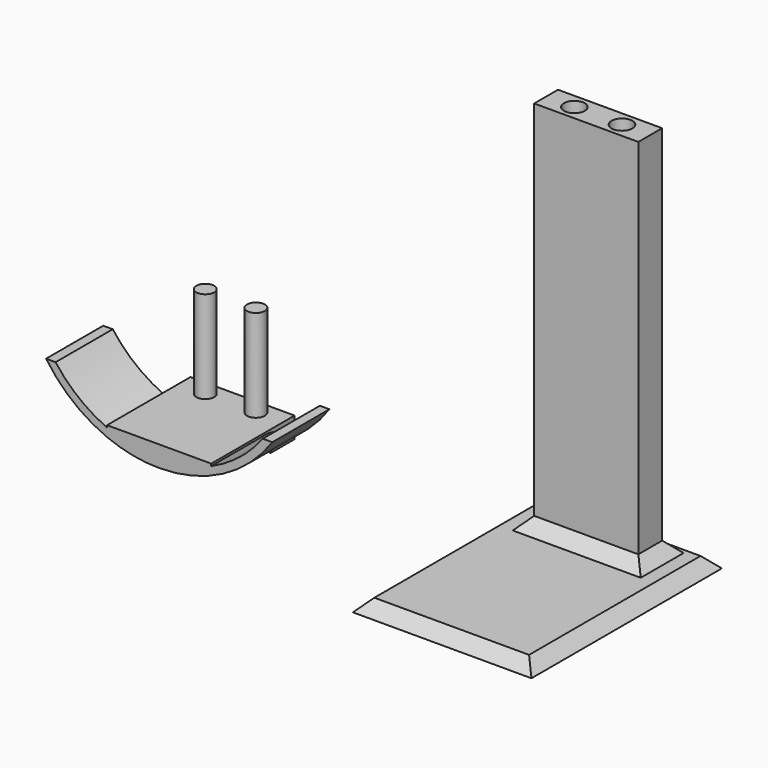
from build123d import *

# Parameters (mm, degrees)
F0_W      = 76.2
F0_H      = 101.6
F0_W_2    = 44.45
F0_H_2    = 12.7
F1_DEPTH  = 5.08
F2_DEPTH  = 165.1
F3_R      = 4.445
F4_DEPTH  = 50.8
F5_W      = 44.45
F5_H      = 12.7
F5_R      = 3.81
F6_DEPTH  = 8.89
F7_DEPTH  = 48.26
F9_DEPTH  = 31.75
F10_DEPTH = 1.27
F11_SIZE  = 5.07999


# Not quite as in the source:
# - a fillet or chamfer is up to 0.001 mm smaller than in the source, because OpenCascade refuses the exact size


with BuildPart() as f1:
    # F0 (on Top) → F1 (new body)
    with BuildSketch(Plane.XY):
        Rectangle(F0_W, F0_H)
        with Locations((0, 32.4159748852)):
            Rectangle(F0_W_2, F0_H_2, mode=Mode.SUBTRACT)
    extrude(amount=F1_DEPTH)

    # F0 (on Top) → F2 (join)
    with BuildSketch(Plane.XY):
        with Locations((0, 32.4159748852)):
            Rectangle(F0_W_2, F0_H_2)
    extrude(amount=F2_DEPTH)

    # F3 (on face) → F4 (cut)
    with BuildSketch(Plane.XY.offset(165.1)):
        with Locations((-10.16, 32.4159748852)):
            Circle(F3_R)
        with Locations((10.16, 32.4159748852)):
            Circle(F3_R)
    extrude(amount=-F4_DEPTH, mode=Mode.SUBTRACT)

    # F11 (size 5.08 in the source; OpenCascade refuses exactly that, so slightly less here)
    f11_edges = [f1.edges().sort_by_distance(p)[0] for p in [
        (38.1, 0, 5.08),
        (0, 50.8, 5.08),
        (-38.1, 0, 5.08),
        (0, -50.8, 5.08),
        (22.225, 32.415975, 5.08),
        (0, 26.065975, 5.08),
        (-22.225, 32.415975, 5.08),
        (0, 38.765975, 5.08),
    ]]
    chamfer(f11_edges, length=F11_SIZE)


with BuildPart() as f6:
    # F5 (on Top) → F6 (new body)
    with BuildSketch(Plane.XY):
        with Locations((-153.5560860872, 28.2728751957)):
            Rectangle(F5_W, F5_H)
        with Locations((-164.3510860872, 28.2728751957)):
            Circle(F5_R, mode=Mode.SUBTRACT)
        with Locations((-142.7610860872, 28.2728751957)):
            Circle(F5_R, mode=Mode.SUBTRACT)
    extrude(amount=F6_DEPTH)

    # F5 (on Top) → F7 (join)
    with BuildSketch(Plane.XY):
        with Locations((-164.3510860872, 28.2728751957)):
            Circle(F5_R)
        with Locations((-142.7610860872, 28.2728751957)):
            Circle(F5_R)
    extrude(amount=F7_DEPTH)

    # F8 (on face) → F9 (join)
    with BuildSketch(Plane.XZ.offset(-21.9228751957)):
        with BuildLine():
            Line((-175.7810860872, 7.9697383106), (-175.7810860872, 4.3824305473))
            ThreePointArc((-175.7810860872, 4.3824305473), (-164.8825631117, 1.1060553071), (-153.5560861917, 0))
            ThreePointArc((-153.5560861917, 0), (-142.2296091652, 1.1060552869), (-131.3310860872, 4.3824305473))
            Line((-131.3310860872, 4.3824305473), (-131.3310860872, 7.9697383106))
            ThreePointArc((-131.3310860872, 7.9697383106), (-153.5560860872, 3.302), (-175.7810860872, 7.9697383106))
        make_face()
        with BuildLine():
            Line((-105.2960860872, 25.4), (-109.3600860872, 25.4))
            ThreePointArc((-109.3600860872, 25.4), (-119.2211066073, 15.2674527622), (-131.3310860872, 7.9697383106))
            Line((-131.3310860872, 7.9697383106), (-131.3310860872, 4.3824305473))
            ThreePointArc((-131.3310860872, 4.3824305473), (-116.7801651243, 12.9917275683), (-105.2960860872, 25.4))
        make_face()
        with BuildLine():
            Line((-197.7520860872, 25.4), (-201.8160860872, 25.4))
            ThreePointArc((-201.8160860872, 25.4), (-190.3320070502, 12.9917275683), (-175.7810860872, 4.3824305473))
            Line((-175.7810860872, 4.3824305473), (-175.7810860872, 7.9697383106))
            ThreePointArc((-175.7810860872, 7.9697383106), (-187.8910655672, 15.2674527622), (-197.7520860872, 25.4))
        make_face()
        with BuildLine():
            Line((-175.7810860872, 8.89), (-175.7810860872, 7.9697383106))
            ThreePointArc((-175.7810860872, 7.9697383106), (-153.5560860872, 3.302), (-131.3310860872, 7.9697383106))
            Line((-131.3310860872, 7.9697383106), (-131.3310860872, 8.89))
            Line((-131.3310860872, 8.89), (-175.7810860872, 8.89))
        make_face()
    extrude(amount=F9_DEPTH)

    # F10 (cut): faces of the model
    f10_faces = [f6.faces().sort_by_distance(p)[0] for p in [
        (-118.407316074, 21.9228751957, 14.6525302176),
        (-188.7048561005, 21.9228751957, 14.6525302176),
    ]]
    extrude(f10_faces, amount=-F10_DEPTH, mode=Mode.SUBTRACT)


solid = Compound([f1.part, f6.part])
